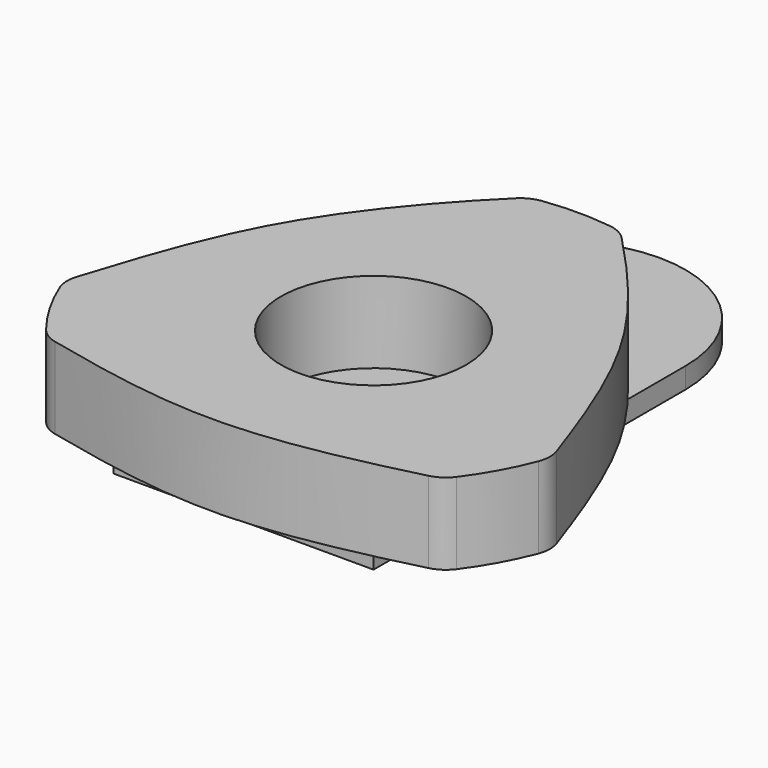
from build123d import *

# Parameters (mm, degrees)
F2_DEPTH  = 25
F0_R      = 28.5
F3_DEPTH  = 25
F4_R      = 1.9
F4_R_2    = 16.3
F5_DEPTH  = 2
F7_DEPTH  = 6.4
F13_R     = 3.85
F14_DEPTH = 25
F15_R     = 1.9
F15_W     = 8
F15_H     = 16
F16_DEPTH = 25
F15_R_2   = 3.1
F17_DEPTH = 25


with BuildPart() as f2:
    # F1 (on Top) → F2 (new body)
    with BuildSketch(Plane.XY):
        with BuildLine():
            add(Edge.make_bspline(
                [(-73.1789692579, -22.7385899679), (-67.4229557867, -4.6103998422), (-55.9062049057, 31.3935288647), (-29.1523327535, 62.4691751234), (-16.2776546186, 75.1598383007)],
                knots=[0.0300459098, 0.0300459098, 0.0300459098, 0.0300459098, 0.4991892343, 0.971612758, 0.971612758, 0.971612758, 0.971612758], degree=3))
            ThreePointArc((-73.1789692579, -22.7385899679), (-73.6404359954, -26.1507340498), (-72.9172177651, -29.5171318541))
            ThreePointArc((-72.9172177651, -29.5171318541), (-68.0180262426, -39.5187275297), (-61.7555025142, -48.7282220969))
            ThreePointArc((-61.7555025142, -48.7282220969), (-59.2584349201, -50.9802076446), (-56.1560727225, -52.2771788358))
            add(Edge.make_bspline(
                [(-56.1560727225, -52.2771788358), (-37.4626070784, -56.5959409061), (0.0447461414, -64.2042541394), (38.5139105355, -55.4955216989), (57.5112062949, -50.7122802135)],
                knots=[0.0288892767, 0.0288892767, 0.0288892767, 0.0288892767, 0.4970222039, 0.9722377077, 0.9722377077, 0.9722377077, 0.9722377077], degree=3))
            ThreePointArc((57.5112062949, -50.7122802135), (60.6219456552, -49.3318528918), (63.0895920344, -46.9881378269))
            ThreePointArc((63.0895920344, -46.9881378269), (68.8652506753, -38.0231372842), (73.3752696435, -28.3593286989))
            ThreePointArc((73.3752696435, -28.3593286989), (74.0462704517, -24.9237404958), (73.4920964317, -21.467384099))
            add(Edge.make_bspline(
                [(16.3087167239, 74.9895741586), (29.3830090096, 61.3889009081), (54.2893459649, 32.8352732382), (67.2195004815, -3.4438955282), (73.4920964317, -21.467384099)],
                knots=[0.0280155618, 0.0280155618, 0.0280155618, 0.0280155618, 0.4979163288, 0.9708005249, 0.9708005249, 0.9708005249, 0.9708005249], degree=3))
            ThreePointArc((16.3087167239, 74.9895741586), (13.6196421952, 76.9795063508), (10.4247227385, 77.9711925991))
            ThreePointArc((10.4247227385, 77.9711925991), (-0.0914096856, 78.6649436774), (-10.6059014171, 77.9467547409))
            ThreePointArc((-10.6059014171, 77.9467547409), (-13.6677134751, 77.0131058407), (-16.2776546186, 75.1598383007))
        make_face()
    extrude(amount=F2_DEPTH)

    # F0 (on Top) → F3 (cut)
    with BuildSketch(Plane.XY):
        Circle(F0_R)
    extrude(amount=F3_DEPTH, mode=Mode.SUBTRACT)


with BuildPart() as f5:
    # F4 (on Top) → F5 (new body)
    with BuildSketch(Plane.XY):
        with BuildLine():
            Line((-31, -38), (31, -38))
            ThreePointArc((31, -38), (35.9497474683, -35.9497474683), (38, -31))
            Line((38, -31), (38, 31))
            ThreePointArc((38, 31), (35.9497474683, 35.9497474683), (31, 38))
            Line((31, 38), (-31, 38))
            ThreePointArc((-31, 38), (-35.9497474683, 35.9497474683), (-38, 31))
            Line((-38, 31), (-38, -31))
            ThreePointArc((-38, -31), (-35.9497474683, -35.9497474683), (-31, -38))
        make_face()
        with Locations((-32.4, -32.4)):
            Circle(F4_R, mode=Mode.SUBTRACT)
        with Locations((32.4, -32.4)):
            Circle(F4_R, mode=Mode.SUBTRACT)
        with Locations((-32.4, 32.4)):
            Circle(F4_R, mode=Mode.SUBTRACT)
        Circle(F4_R_2, mode=Mode.SUBTRACT)
        with Locations((32.4, 32.4)):
            Circle(F4_R, mode=Mode.SUBTRACT)
    extrude(amount=F5_DEPTH)


with BuildPart() as f7:
    # F6 (on Top) → F7 (new body)
    with BuildSketch(Plane.XY):
        with BuildLine():
            Line((-40, -80), (40, -80))
            Line((40, -80), (40, 40))
            ThreePointArc((40, 40), (28.2842712475, 68.2842712475), (0, 80))
            ThreePointArc((0, 80), (-28.2842712475, 68.2842712475), (-40, 40))
            Line((-40, 40), (-40, -80))
        make_face()
    extrude(amount=F7_DEPTH)


with BuildPart() as f7_1:
    # F8: moved
    add(f7.part.moved(Location((0, 0, -6.4))))


with BuildPart() as f7_2:
    # F9: moved
    add(f7_1.part.moved(Location((0, 40, 0))))


with BuildPart() as f5_1:
    # F10: moved
    add(f5.part.moved(Location((0, 0, -2))))


with BuildPart() as f5_2:
    # F11: moved
    add(f5_1.part.moved(Location((0, 0, -6.4))))


with BuildPart() as f7_3:
    # F12: moved
    add(f7_2.part.moved(Location((0, -10, 0))))

    # F13 (on Top) → F14 (cut)
    with BuildSketch(Plane.XY):
        with Locations((0, 88)):
            Circle(F13_R)
    extrude(amount=-F14_DEPTH, mode=Mode.SUBTRACT)

    # F15 (on face) → F16 (cut)
    with BuildSketch(Plane(origin=(0, 0, -6.4), x_dir=(1, 0, 0), z_dir=(0, 0, -1))):
        with Locations((-32.4, 32.4)):
            Circle(F15_R)
        with Locations((32.4, 32.4)):
            Circle(F15_R)
        with Locations((32.4, -32.4)):
            Circle(F15_R)
        with Locations((-32.4, -32.4)):
            Circle(F15_R)
        with Locations((15, 0)):
            Rectangle(F15_W, F15_H)
    extrude(amount=-F16_DEPTH, mode=Mode.SUBTRACT)

    # F15 (on face) → F17 (cut)
    with BuildSketch(Plane(origin=(0, 0, -6.4), x_dir=(1, 0, 0), z_dir=(0, 0, -1))):
        Circle(F15_R_2)
    extrude(amount=-F17_DEPTH, mode=Mode.SUBTRACT)


solid = Compound([f2.part, f5_2.part, f7_3.part])
